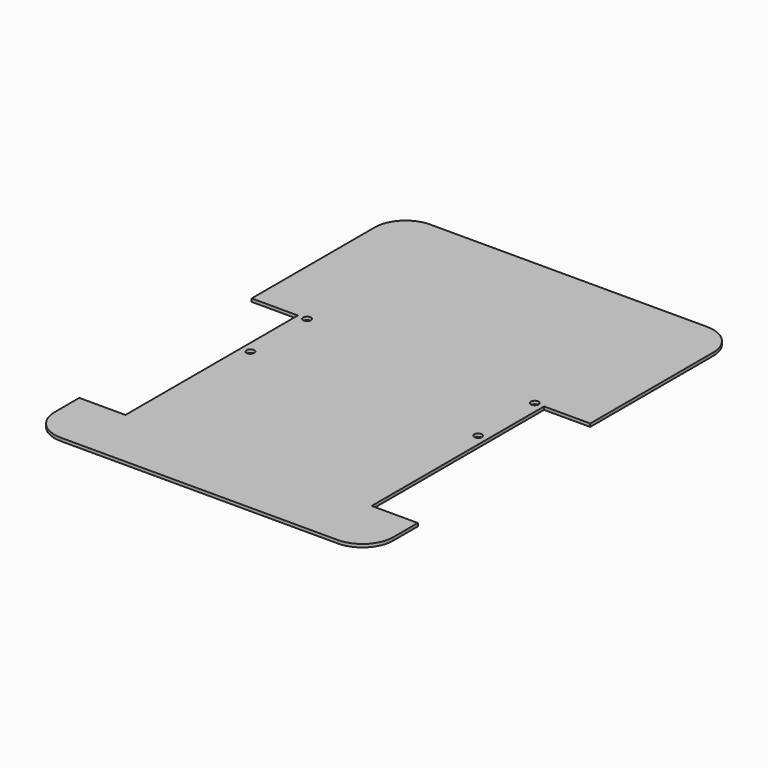
from build123d import *

# Parameters (mm, degrees)
F1_DEPTH = 1
F3_D     = 2.5


# Not quite as in the source:
# - a feature names something its author has since deleted; it is built from what else it names


with BuildPart() as f1:
    # F0 (on Top) → F1 (new body)
    with BuildSketch(Plane.XY):
        with BuildLine():
            Line((45, 0), (-45, 0))
            ThreePointArc((-45, 0), (-52.0710678119, -2.9289321881), (-55, -10))
            Line((-55, -10), (-55, -60))
            Line((-55, -60), (-40, -60))
            Line((-40, -60), (-40, -130))
            Line((-40, -130), (-55, -130))
            Line((-55, -130), (-55, -140))
            ThreePointArc((-55, -140), (-52.0710678119, -147.0710678119), (-45, -150))
            Line((-45, -150), (45, -150))
            ThreePointArc((45, -150), (52.0710678119, -147.0710678119), (55, -140))
            Line((55, -140), (55, -130))
            Line((55, -130), (40, -130))
            Line((40, -130), (40, -60))
            Line((40, -60), (55, -60))
            Line((55, -60), (55, -10))
            ThreePointArc((55, -10), (52.0710678119, -2.9289321881), (45, 0))
        make_face()
    extrude(amount=F1_DEPTH)

    # F3 (through all)
    with Locations(Plane.XY.offset(1)):
        with Locations((37, -60), (37, -83), (-37, -60), (-37, -83)):
            Hole(F3_D / 2)


solid = f1.part
